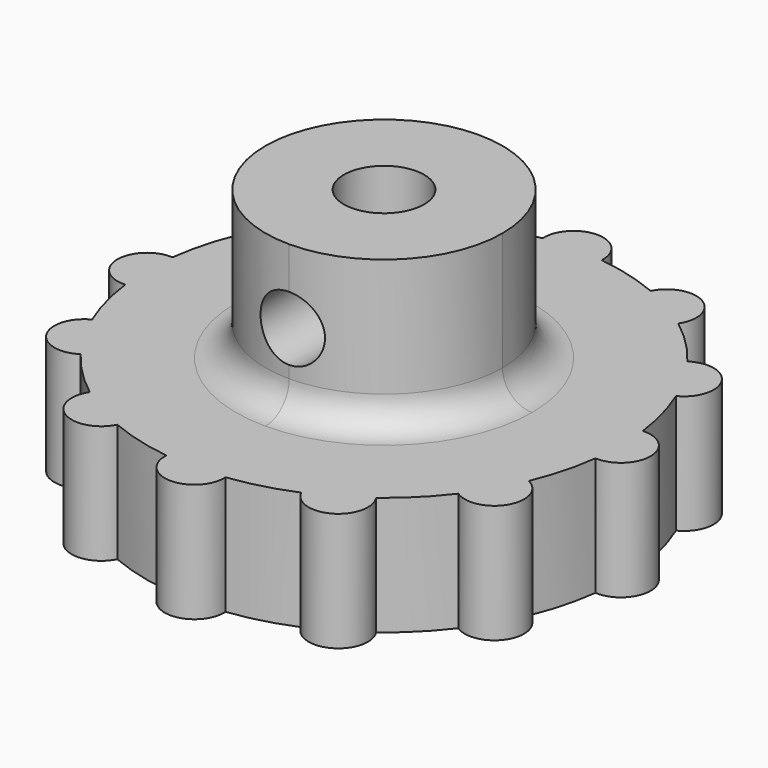
from build123d import *

# Parameters (mm, degrees)
F0_R         = 12.7
F1_DEPTH     = 6.35
F3_DEPTH     = 3.175
F4_W         = 12.7
F4_H         = 12.7
F5_DEPTH     = 7.9375
F7_DEPTH     = 6.35
F8_COUNT     = 12
F8_ANGLE     = 330
F9_R         = 2.15265
F10_DEPTH    = 11.1125
F11_R        = 1.7272
F12_REACH    = 25.5237593299
F13_T1_DEPTH = 7.9375
F14_R        = 1.5875


# Not quite as in the source:
# - a fillet or chamfer that OpenCascade refuses, or shapes differently, is made with other operations: its cross-section is extruded or revolved along the edge and cut away or added


with BuildPart() as f1:
    # F0 (on Top) → F1 (new body)
    with BuildSketch(Plane.XY):
        Circle(F0_R)
    extrude(amount=F1_DEPTH)

    # F2 (on face) → F3 (cut)
    with BuildSketch(Plane(origin=(0, 0, 0), x_dir=(1, 0, 0), z_dir=(0, 0, -1))):
        Polygon((2.6100007461, 4.5206539), (-2.6100007461, 4.5206539), (-5.2200014922, 0), (-2.6100007461, -4.5206539), (2.6100007461, -4.5206539), (5.2200014922, 0), align=None)
    extrude(amount=-F3_DEPTH, mode=Mode.SUBTRACT)

    # F4 (on face) → F5 (join)
    with BuildSketch(Plane.XY.offset(6.35)):
        Rectangle(F4_W, F4_H)
    extrude(amount=F5_DEPTH)

    # F6 (on face) → F7 (join, through all)
    with BuildSketch(Plane(origin=(0, 0, 0), x_dir=(1, 0, 0), z_dir=(0, 0, -1))):
        with BuildLine():
            ThreePointArc((-1.5843963802, 12.60078125), (0, 12.7), (1.5843963802, 12.60078125))
            ThreePointArc((1.5843963802, 12.60078125), (0, 14.2875), (-1.5843963802, 12.60078125))
        make_face()
    f7 = extrude(amount=-F7_DEPTH)

    # F8: F7 ×12 about axis
    f8_axis = Axis((0, 0, 0), (0, 0, -1))
    for i in range(1, F8_COUNT):
        add(f7.rotate(f8_axis, i * F8_ANGLE / (F8_COUNT - 1)))

    # F9 (on face) → F10 (cut, through all)
    with BuildSketch(Plane(origin=(0, 0, 3.175), x_dir=(1, 0, 0), z_dir=(0, 0, -1))):
        Circle(F9_R)
    extrude(amount=-F10_DEPTH, mode=Mode.SUBTRACT)

    f12_end = f1.faces().sort_by_distance((-2.15265, 0, 8.73125))[0]
    # F11 (on face) → F12 (cut, up to a face of the model that its end follows)
    with BuildSketch(Plane.XZ.offset(6.35)):
        with Locations((0, 10.31875)):
            Circle(F11_R)
    f12_long = extrude(amount=-F12_REACH, mode=Mode.PRIVATE)
    add(split(f12_long, bisect_by=f12_end, keep=Keep.ALL, mode=Mode.PRIVATE).solids().sort_by_distance((0, -6.35, 10.31875))[0], mode=Mode.SUBTRACT)

    # F13: fillet of radius 6.35 on 4 edges, made by hand

    # F13_s2 → F13_t1 (cut)
    with BuildSketch(Plane.XY.offset(6.35)):
        with BuildLine():
            ThreePointArc((0, -6.35), (-4.4901280605, -4.4901280605), (-6.35, 0))
            Line((-6.35, 0), (-6.477, 0))
            Line((-6.477, 0), (-6.477, -6.477))
            Line((-6.477, -6.477), (0, -6.477))
            Line((0, -6.477), (0, -6.35))
        make_face()
        with BuildLine():
            ThreePointArc((6.35, 0), (4.4901280605, -4.4901280605), (0, -6.35))
            Line((0, -6.35), (0, -6.477))
            Line((0, -6.477), (6.477, -6.477))
            Line((6.477, -6.477), (6.477, 0))
            Line((6.477, 0), (6.35, 0))
        make_face()
        with BuildLine():
            ThreePointArc((6.35, 0), (4.4901280605, 4.4901280605), (0, 6.35))
            Line((0, 6.35), (0, 6.477))
            Line((0, 6.477), (6.477, 6.477))
            Line((6.477, 6.477), (6.477, 0))
            Line((6.477, 0), (6.35, 0))
        make_face()
        with BuildLine():
            ThreePointArc((-6.35, 0), (-4.4901280605, 4.4901280605), (0, 6.35))
            Line((0, 6.35), (0, 6.477))
            Line((0, 6.477), (-6.477, 6.477))
            Line((-6.477, 6.477), (-6.477, 0))
            Line((-6.477, 0), (-6.35, 0))
        make_face()
    extrude(amount=F13_T1_DEPTH, mode=Mode.SUBTRACT)

    # F14
    f14_edges = [f1.edges().sort_by_distance(p)[0] for p in [
        (4.490128, 4.490128, 6.35),
    ]]
    fillet(f14_edges, radius=F14_R)


solid = f1.part
